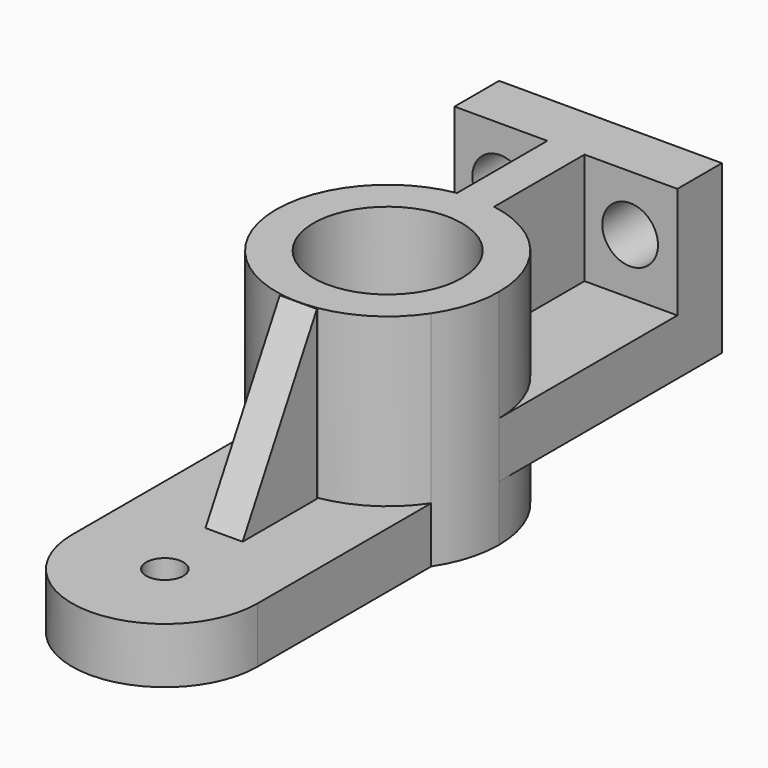
from build123d import *

# Parameters (mm, degrees)
F0_R      = 20
F1_DEPTH  = 60
F0_R_2    = 5
F2_DEPTH  = 15
F3_DEPTH  = 60
F4_DEPTH  = 45
F5_DEPTH  = 15
F7_DEPTH  = 30
F9_DEPTH  = 5
F10_R     = 7.5
F11_DEPTH = 15


with BuildPart() as f1:
    # F0 (on Top) → F1 (new body)
    with BuildSketch(Plane.XY):
        with BuildLine():
            ThreePointArc((25, -16.5831239518), (28.7228132327, -8.6602540378), (30, 0))
            ThreePointArc((30, 0), (22.9128784748, 19.364916731), (5, 29.5803989155))
            ThreePointArc((5, 29.5803989155), (0, 30), (-5, 29.5803989155))
            ThreePointArc((-5, 29.5803989155), (-22.9128784748, 19.364916731), (-30, 0))
            ThreePointArc((-30, 0), (-28.7228132327, -8.6602540378), (-25, -16.5831239518))
            ThreePointArc((-25, -16.5831239518), (-16.3472410247, -25.1548744954), (-5, -29.5803989155))
            ThreePointArc((-5, -29.5803989155), (0, -30), (5, -29.5803989155))
            ThreePointArc((5, -29.5803989155), (16.3472410247, -25.1548744954), (25, -16.5831239518))
        make_face()
        Circle(F0_R, mode=Mode.SUBTRACT)
    extrude(amount=F1_DEPTH)

    # F0 (on Top) → F2 (join)
    with BuildSketch(Plane.XY):
        with BuildLine():
            Line((25, -75), (25, -16.5831239518))
            ThreePointArc((25, -16.5831239518), (16.3472410247, -25.1548744954), (5, -29.5803989155))
            Line((5, -29.5803989155), (5, -54.5803989155))
            Line((5, -54.5803989155), (0, -54.5803989155))
            Line((0, -54.5803989155), (-5, -54.5803989155))
            Line((-5, -54.5803989155), (-5, -29.5803989155))
            ThreePointArc((-5, -29.5803989155), (-16.3472410247, -25.1548744954), (-25, -16.5831239518))
            Line((-25, -16.5831239518), (-25, -75))
            ThreePointArc((-25, -75), (0, -100), (25, -75))
        make_face()
        with Locations((0, -75)):
            Circle(F0_R_2, mode=Mode.SUBTRACT)
        with BuildLine():
            Line((5, -54.5803989155), (5, -29.5803989155))
            ThreePointArc((5, -29.5803989155), (0, -30), (-5, -29.5803989155))
            Line((-5, -29.5803989155), (-5, -54.5803989155))
            Line((-5, -54.5803989155), (0, -54.5803989155))
            Line((0, -54.5803989155), (5, -54.5803989155))
        make_face()
    extrude(amount=F2_DEPTH)

    # F0 (on Top) → F3 (join)
    with BuildSketch(Plane.XY):
        with BuildLine():
            ThreePointArc((-30, 0), (-22.9128784748, 19.364916731), (-5, 29.5803989155))
            Line((-5, 29.5803989155), (-5, 60))
            Line((-5, 60), (-30, 60))
            Line((-30, 60), (-30, 0))
        make_face()
        with BuildLine():
            ThreePointArc((-5, 29.5803989155), (0, 30), (5, 29.5803989155))
            Line((5, 29.5803989155), (5, 60))
            Line((5, 60), (30, 60))
            Line((30, 60), (30, 75))
            Line((30, 75), (-30, 75))
            Line((-30, 75), (-30, 60))
            Line((-30, 60), (-5, 60))
            Line((-5, 60), (-5, 29.5803989155))
        make_face()
        with BuildLine():
            ThreePointArc((5, 29.5803989155), (22.9128784748, 19.364916731), (30, 0))
            Line((30, 0), (30, 60))
            Line((30, 60), (5, 60))
            Line((5, 60), (5, 29.5803989155))
        make_face()
    extrude(amount=F3_DEPTH)

    # F0 (on Top) → F4 (join)
    with BuildSketch(Plane.XY):
        with BuildLine():
            ThreePointArc((25, -16.5831239518), (28.7228132327, -8.6602540378), (30, 0))
            ThreePointArc((30, 0), (22.9128784748, 19.364916731), (5, 29.5803989155))
            ThreePointArc((5, 29.5803989155), (0, 30), (-5, 29.5803989155))
            ThreePointArc((-5, 29.5803989155), (-22.9128784748, 19.364916731), (-30, 0))
            ThreePointArc((-30, 0), (-28.7228132327, -8.6602540378), (-25, -16.5831239518))
            ThreePointArc((-25, -16.5831239518), (-16.3472410247, -25.1548744954), (-5, -29.5803989155))
            ThreePointArc((-5, -29.5803989155), (0, -30), (5, -29.5803989155))
            ThreePointArc((5, -29.5803989155), (16.3472410247, -25.1548744954), (25, -16.5831239518))
        make_face()
        Circle(F0_R, mode=Mode.SUBTRACT)
        with BuildLine():
            ThreePointArc((-5, 29.5803989155), (0, 30), (5, 29.5803989155))
            Line((5, 29.5803989155), (5, 60))
            Line((5, 60), (30, 60))
            Line((30, 60), (30, 75))
            Line((30, 75), (-30, 75))
            Line((-30, 75), (-30, 60))
            Line((-30, 60), (-5, 60))
            Line((-5, 60), (-5, 29.5803989155))
        make_face()
    extrude(amount=F4_DEPTH)

    # F0 (on Top) → F5 (cut)
    with BuildSketch(Plane.XY):
        with BuildLine():
            ThreePointArc((-30, 0), (-22.9128784748, 19.364916731), (-5, 29.5803989155))
            Line((-5, 29.5803989155), (-5, 60))
            Line((-5, 60), (-30, 60))
            Line((-30, 60), (-30, 0))
        make_face()
        with BuildLine():
            ThreePointArc((-5, 29.5803989155), (0, 30), (5, 29.5803989155))
            Line((5, 29.5803989155), (5, 60))
            Line((5, 60), (30, 60))
            Line((30, 60), (30, 75))
            Line((30, 75), (-30, 75))
            Line((-30, 75), (-30, 60))
            Line((-30, 60), (-5, 60))
            Line((-5, 60), (-5, 29.5803989155))
        make_face()
        with BuildLine():
            ThreePointArc((5, 29.5803989155), (22.9128784748, 19.364916731), (30, 0))
            Line((30, 0), (30, 60))
            Line((30, 60), (5, 60))
            Line((5, 60), (5, 29.5803989155))
        make_face()
    extrude(amount=F5_DEPTH, mode=Mode.SUBTRACT)

    # F6 (on face) → F7 (cut)
    with BuildSketch(Plane.XY.offset(60)):
        with BuildLine():
            Line((-5, 29.5803989155), (-5, 60))
            Line((-5, 60), (-30, 60))
            Line((-30, 60), (-30, 0))
            ThreePointArc((-30, 0), (-22.9128784748, 19.364916731), (-5, 29.5803989155))
        make_face()
        with BuildLine():
            Line((5, 60), (5, 29.5803989155))
            ThreePointArc((5, 29.5803989155), (22.9128784748, 19.364916731), (30, 0))
            Line((30, 0), (30, 60))
            Line((30, 60), (5, 60))
        make_face()
    extrude(amount=-F7_DEPTH, mode=Mode.SUBTRACT)

    # F8 (on Right) → F9 (join, symmetric)
    with BuildSketch(Plane.YZ):
        Polygon((-55.0730913877, 15), (-30.0730913877, 15), (-30.0730913877, 60), align=None)
    extrude(amount=F9_DEPTH, both=True)

    # F10 (on face) → F11 (cut)
    with BuildSketch(Plane.XZ.offset(-60)):
        with Locations((-17.7129209042, 45)):
            Circle(F10_R)
        with Locations((17.2870790958, 45)):
            Circle(F10_R)
    extrude(amount=-F11_DEPTH, mode=Mode.SUBTRACT)


solid = f1.part
